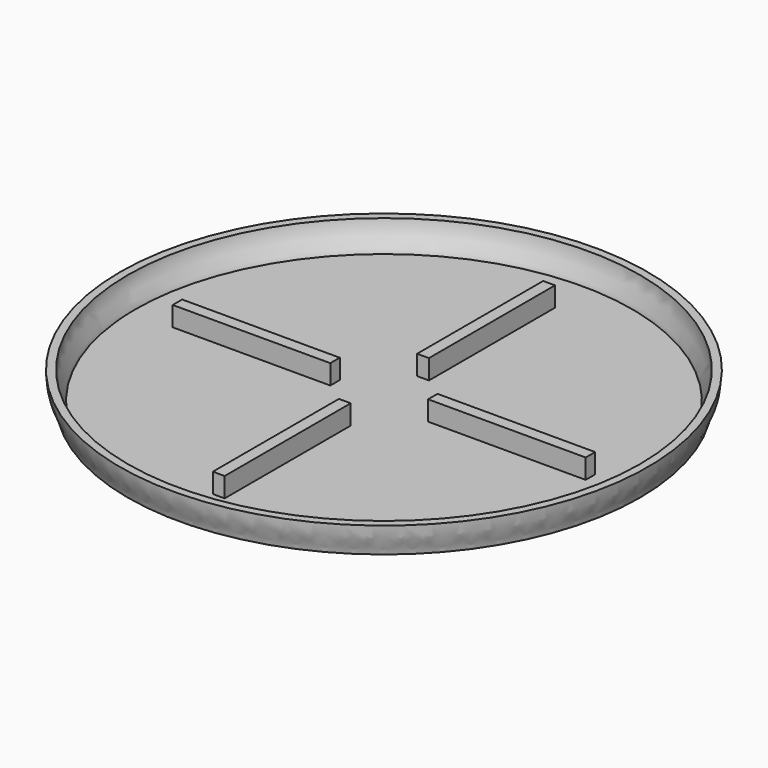
from build123d import *

# Parameters (mm, degrees)
F0_R     = 130
F0_R_2   = 126
F3_DEPTH = 1
F4_W     = 6
F4_H     = 80
F4_W_2   = 80
F4_H_2   = 6
F5_DEPTH = 10


with BuildPart() as f2:
    # F1 (on Front) → F2 (revolve)
    with BuildSketch(Plane.XZ):
        with BuildLine():
            Line((-130, 0), (-126, 0))
            add(Edge.make_bspline(
                [(-126, 0), (-126, 5.4461690597), (-130, 7.5), (-130, 15)],
                knots=[0, 0, 0, 0, 15.5241746963, 15.5241746963, 15.5241746963, 15.5241746963], degree=3))
            Line((-130, 15), (-134, 15))
            add(Edge.make_bspline(
                [(-130, 0), (-130, 0.4359507241), (-130.0760614447, 1.1849617929), (-130.3656491399, 2.2419075402), (-130.8735212704, 3.4664092667), (-131.6006899037, 4.9719563522), (-132.4517866219, 6.8319482048), (-133.2625447424, 9.1028083194), (-133.8503819176, 11.8027229937), (-134, 13.8847222222), (-134, 15)],
                knots=[0, 0, 0, 0, 0.125, 0.25, 0.375, 0.5, 0.625, 0.75, 0.875, 1, 1, 1, 1], degree=3))
        make_face()
    revolve(axis=Axis((0, 0, 15.9704145044), (0, 0, 1)))

    # F0 (on Top) → F3 (join)
    with BuildSketch(Plane.XY):
        Circle(F0_R)
        Circle(F0_R_2, mode=Mode.SUBTRACT)
        Circle(F0_R_2)
    extrude(amount=F3_DEPTH)

    # F4 (on face) → F5 (join)
    with BuildSketch(Plane.XY.offset(1)):
        with Locations((0, 64.819347292)):
            Rectangle(F4_W, F4_H)
        with Locations((-64.819347292, 0)):
            Rectangle(F4_W_2, F4_H_2)
        with Locations((64.819347292, 0)):
            Rectangle(F4_W_2, F4_H_2)
        with Locations((0, -64.819347292)):
            Rectangle(F4_W, F4_H)
    extrude(amount=F5_DEPTH)


solid = f2.part
